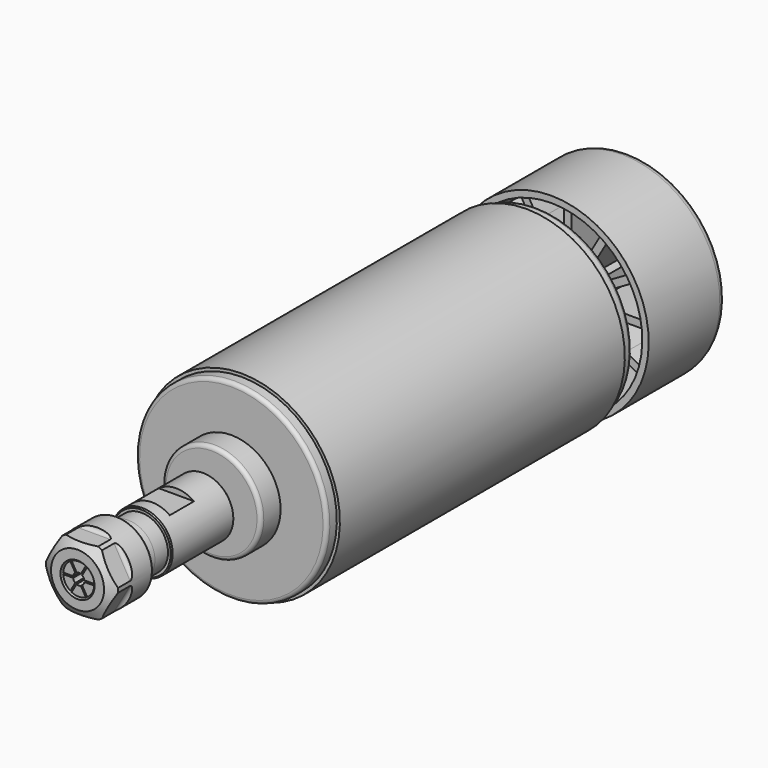
from build123d import *

# Parameters (mm, degrees)
F0_W      = 2.5
F0_H      = 4
F2_R      = 2
F3_R      = 1
F4_SIZE   = 1
F6_W      = 8
F6_H      = 2.5
F7_DEPTH  = 12.5
F10_R     = 0.5
F13_R     = 12
F14_DEPTH = 6.5
F15_R     = 0.99999
F16_R     = 4.5
F17_DEPTH = 0.4
F18_R     = 4.5
F19_DEPTH = 3
F21_DEPTH = 20
F23_DEPTH = 16.5


# Not quite as in the source:
# - a fillet or chamfer that OpenCascade refuses, or shapes differently, is made with other operations: its cross-section is extruded or revolved along the edge and cut away or added
# - a fillet or chamfer is up to 0.001 mm smaller than in the source, because OpenCascade refuses the exact size


with BuildPart() as f1:
    # F0 (on Right) → F1 (revolve)
    with BuildSketch(Plane.YZ):
        Polygon((-68.75, 4), (-68.75, 0), (68.75, 0), (68.75, 4), (65.25, 4), (65.25, 17.25), (68.75, 17.25), (68.75, 25.75), (43.29, 25.75), (43.29, 24.05), (48.75, 24.05), (48.75, 4), (44.93, 4), (44.93, 13), (38.39, 13), (38.39, 25.2), (35.09, 25.2), (35.09, 26), (-58.91, 26), (-58.91, 25.2), (-62.21, 25.2), (-62.21, 13), (-68.75, 13), align=None)
        with Locations((-70, 2)):
            Rectangle(F0_W, F0_H)
        Polygon((-106.25, 0), (-71.25, 0), (-71.25, 4), (-71.25, 8), (-91.85, 8), (-91.85, 7), (-96.15, 7), (-106.25, 6.75), align=None)
    revolve(axis=Axis((0, -2.606525797, 0), (0, 1, 0)))

    # F2
    f2_edges = [f1.edges().sort_by_distance(p)[0] for p in [
        (0, 68.75, -25.75),
    ]]
    fillet(f2_edges, radius=F2_R)

    # F3
    f3_edges = [f1.edges().sort_by_distance(p)[0] for p in [
        (0, 38.39, -25.2),
        (0, -62.21, -25.2),
        (0, -68.75, -13),
        (0, 44.93, -13),
    ]]
    fillet(f3_edges, radius=F3_R)

    # F4
    f4_edges = [f1.edges().sort_by_distance(p)[0] for p in [
        (0, 68.75, -4),
    ]]
    chamfer(f4_edges, length=F4_SIZE)

    # F5: chamfer of 0.3 on 3 edges, made by hand

    # F5_s1 → F5_t2 (revolve, cut)
    with BuildSketch(Plane.YZ):
        Polygon((-71.25, 7.7), (-71.55, 8), (-71.25, 8), align=None)
    revolve(axis=Axis((0, -71.25, 0), (0, 1, 0)), mode=Mode.SUBTRACT)

    # F5_s3 → F5_t4 (revolve, cut)
    with BuildSketch(Plane.YZ):
        Polygon((-91.55, 8), (-91.85, 7.7), (-91.85, 8), align=None)
    revolve(axis=Axis((0, -91.85, 0), (0, 1, 0)), mode=Mode.SUBTRACT)

    # F5_s5 → F5_t6 (revolve, cut)
    with BuildSketch(Plane.YZ):
        Polygon((-105.9574234688, 6.7572419933), (-106.25, 6.4573338539), (-106.25, 6.75), align=None)
    revolve(axis=Axis((0, -106.25, 0), (0, 1, 0)), mode=Mode.SUBTRACT)

    # F6 (on Right) → F7 (cut, symmetric)
    with BuildSketch(Plane.YZ):
        with Locations((-84.35, 7.75)):
            Rectangle(F6_W, F6_H)
        with Locations((-84.35, -7.75)):
            Rectangle(F6_W, F6_H)
    extrude(amount=F7_DEPTH, both=True, mode=Mode.SUBTRACT)

    # F20 (on face) → F21 (cut)
    with BuildSketch(Plane(origin=(0, 65.25, 0), x_dir=(-1, 0, 0), z_dir=(0, 1, 0))):
        with BuildLine():
            ThreePointArc((-5.5, 4.3301270189), (-4.9497474683, 4.9497474683), (-4.3301270189, 5.5))
            Line((-4.3301270189, 5.5), (-9.4765204534, 14.4138149043))
            ThreePointArc((-9.4765204534, 14.4138149043), (-12.1975919755, 12.1975919755), (-14.4138149043, 9.4765204534))
            Line((-14.4138149043, 9.4765204534), (-5.5, 4.3301270189))
        make_face()
        with BuildLine():
            Line((-1, 6.9282032303), (-1, 17.2209900993))
            ThreePointArc((-1, 17.2209900993), (-4.464628528, 16.6622205035), (-7.7444696459, 15.4138149043))
            Line((-7.7444696459, 15.4138149043), (-2.5980762114, 6.5))
            ThreePointArc((-2.5980762114, 6.5), (-1.8117333157, 6.761480784), (-1, 6.9282032303))
        make_face()
        with BuildLine():
            ThreePointArc((7.7444696459, 15.4138149043), (4.464628528, 16.6622205035), (1, 17.2209900993))
            Line((1, 17.2209900993), (1, 6.9282032303))
            ThreePointArc((1, 6.9282032303), (1.8117333157, 6.761480784), (2.5980762114, 6.5))
            Line((2.5980762114, 6.5), (7.7444696459, 15.4138149043))
        make_face()
        with BuildLine():
            Line((-6.5, 2.5980762114), (-15.4138149043, 7.7444696459))
            ThreePointArc((-15.4138149043, 7.7444696459), (-16.6622205035, 4.464628528), (-17.2209900993, 1))
            Line((-17.2209900993, 1), (-6.9282032303, 1))
            ThreePointArc((-6.9282032303, 1), (-6.761480784, 1.8117333157), (-6.5, 2.5980762114))
        make_face()
        with BuildLine():
            Line((-6.9282032303, -1), (-17.2209900993, -1))
            ThreePointArc((-17.2209900993, -1), (-16.6622205035, -4.464628528), (-15.4138149043, -7.7444696459))
            Line((-15.4138149043, -7.7444696459), (-6.5, -2.5980762114))
            ThreePointArc((-6.5, -2.5980762114), (-6.761480784, -1.8117333157), (-6.9282032303, -1))
        make_face()
        with BuildLine():
            Line((-5.5, -4.3301270189), (-14.4138149043, -9.4765204534))
            ThreePointArc((-14.4138149043, -9.4765204534), (-12.1975919755, -12.1975919755), (-9.4765204534, -14.4138149043))
            Line((-9.4765204534, -14.4138149043), (-4.3301270189, -5.5))
            ThreePointArc((-4.3301270189, -5.5), (-4.9497474683, -4.9497474683), (-5.5, -4.3301270189))
        make_face()
        with BuildLine():
            Line((-2.5980762114, -6.5), (-7.7444696459, -15.4138149043))
            ThreePointArc((-7.7444696459, -15.4138149043), (-4.464628528, -16.6622205035), (-1, -17.2209900993))
            Line((-1, -17.2209900993), (-1, -6.9282032303))
            ThreePointArc((-1, -6.9282032303), (-1.8117333157, -6.761480784), (-2.5980762114, -6.5))
        make_face()
        with BuildLine():
            Line((1, -6.9282032303), (1, -17.2209900993))
            ThreePointArc((1, -17.2209900993), (4.464628528, -16.6622205035), (7.7444696459, -15.4138149043))
            Line((7.7444696459, -15.4138149043), (2.5980762114, -6.5))
            ThreePointArc((2.5980762114, -6.5), (1.8117333157, -6.761480784), (1, -6.9282032303))
        make_face()
        with BuildLine():
            Line((4.3301270189, -5.5), (9.4765204534, -14.4138149043))
            ThreePointArc((9.4765204534, -14.4138149043), (12.1975919755, -12.1975919755), (14.4138149043, -9.4765204534))
            Line((14.4138149043, -9.4765204534), (5.5, -4.3301270189))
            ThreePointArc((5.5, -4.3301270189), (4.9497474683, -4.9497474683), (4.3301270189, -5.5))
        make_face()
        with BuildLine():
            Line((6.5, -2.5980762114), (15.4138149043, -7.7444696459))
            ThreePointArc((15.4138149043, -7.7444696459), (16.6622205035, -4.464628528), (17.2209900993, -1))
            Line((17.2209900993, -1), (6.9282032303, -1))
            ThreePointArc((6.9282032303, -1), (6.761480784, -1.8117333157), (6.5, -2.5980762114))
        make_face()
        with BuildLine():
            Line((6.9282032303, 1), (17.2209900993, 1))
            ThreePointArc((17.2209900993, 1), (16.6622205035, 4.464628528), (15.4138149043, 7.7444696459))
            Line((15.4138149043, 7.7444696459), (6.5, 2.5980762114))
            ThreePointArc((6.5, 2.5980762114), (6.761480784, 1.8117333157), (6.9282032303, 1))
        make_face()
        with BuildLine():
            Line((5.5, 4.3301270189), (14.4138149043, 9.4765204534))
            ThreePointArc((14.4138149043, 9.4765204534), (12.1975919755, 12.1975919755), (9.4765204534, 14.4138149043))
            Line((9.4765204534, 14.4138149043), (4.3301270189, 5.5))
            ThreePointArc((4.3301270189, 5.5), (4.9497474683, 4.9497474683), (5.5, 4.3301270189))
        make_face()
    extrude(amount=-F21_DEPTH, mode=Mode.SUBTRACT)

    # F22 (on face) → F23 (cut)
    with BuildSketch(Plane.XZ.offset(-48.75)):
        with BuildLine():
            Line((17.2209900993, 1), (24.0292009855, 1))
            ThreePointArc((24.0292009855, 1), (23.2305161223, 6.2245980347), (21.3098984861, 11.1485750889))
            Line((21.3098984861, 11.1485750889), (15.4138149043, 7.7444696459))
            ThreePointArc((15.4138149043, 7.7444696459), (16.6622205035, 4.464628528), (17.2209900993, 1))
        make_face()
        with BuildLine():
            ThreePointArc((21.3098984861, -11.1485750889), (23.2305161223, -6.2245980347), (24.0292009855, -1))
            Line((24.0292009855, -1), (17.2209900993, -1))
            ThreePointArc((17.2209900993, -1), (16.6622205035, -4.464628528), (15.4138149043, -7.7444696459))
            Line((15.4138149043, -7.7444696459), (21.3098984861, -11.1485750889))
        make_face()
        with BuildLine():
            Line((14.4138149043, 9.4765204534), (20.3098984861, 12.8806258965))
            ThreePointArc((20.3098984861, 12.8806258965), (17.0059180875, 17.0059180875), (12.8806258965, 20.3098984861))
            Line((12.8806258965, 20.3098984861), (9.4765204534, 14.4138149043))
            ThreePointArc((9.4765204534, 14.4138149043), (12.1975919755, 12.1975919755), (14.4138149043, 9.4765204534))
        make_face()
        with BuildLine():
            ThreePointArc((12.8806258965, -20.3098984861), (17.0059180875, -17.0059180875), (20.3098984861, -12.8806258965))
            Line((20.3098984861, -12.8806258965), (14.4138149043, -9.4765204534))
            ThreePointArc((14.4138149043, -9.4765204534), (12.1975919755, -12.1975919755), (9.4765204534, -14.4138149043))
            Line((9.4765204534, -14.4138149043), (12.8806258965, -20.3098984861))
        make_face()
        with BuildLine():
            Line((7.7444696459, 15.4138149043), (11.1485750889, 21.3098984861))
            ThreePointArc((11.1485750889, 21.3098984861), (6.2245980347, 23.2305161223), (1, 24.0292009855))
            Line((1, 24.0292009855), (1, 17.2209900993))
            ThreePointArc((1, 17.2209900993), (4.464628528, 16.6622205035), (7.7444696459, 15.4138149043))
        make_face()
        with BuildLine():
            ThreePointArc((1, -24.0292009855), (6.2245980347, -23.2305161223), (11.1485750889, -21.3098984861))
            Line((11.1485750889, -21.3098984861), (7.7444696459, -15.4138149043))
            ThreePointArc((7.7444696459, -15.4138149043), (4.464628528, -16.6622205035), (1, -17.2209900993))
            Line((1, -17.2209900993), (1, -24.0292009855))
        make_face()
        with BuildLine():
            ThreePointArc((1, -17.2209900993), (4.464628528, -16.6622205035), (7.7444696459, -15.4138149043))
            Line((7.7444696459, -15.4138149043), (2.5980762114, -6.5))
            ThreePointArc((2.5980762114, -6.5), (1.8117333157, -6.761480784), (1, -6.9282032303))
            Line((1, -6.9282032303), (1, -17.2209900993))
        make_face()
        with BuildLine():
            Line((-1, 17.2209900993), (-1, 24.0292009855))
            ThreePointArc((-1, 24.0292009855), (-6.2245980347, 23.2305161223), (-11.1485750889, 21.3098984861))
            Line((-11.1485750889, 21.3098984861), (-7.7444696459, 15.4138149043))
            ThreePointArc((-7.7444696459, 15.4138149043), (-4.464628528, 16.6622205035), (-1, 17.2209900993))
        make_face()
        with BuildLine():
            ThreePointArc((-11.1485750889, -21.3098984861), (-6.2245980347, -23.2305161223), (-1, -24.0292009855))
            Line((-1, -24.0292009855), (-1, -17.2209900993))
            ThreePointArc((-1, -17.2209900993), (-4.464628528, -16.6622205035), (-7.7444696459, -15.4138149043))
            Line((-7.7444696459, -15.4138149043), (-11.1485750889, -21.3098984861))
        make_face()
        with BuildLine():
            Line((-1, 6.9282032303), (-1, 17.2209900993))
            ThreePointArc((-1, 17.2209900993), (-4.464628528, 16.6622205035), (-7.7444696459, 15.4138149043))
            Line((-7.7444696459, 15.4138149043), (-2.5980762114, 6.5))
            ThreePointArc((-2.5980762114, 6.5), (-1.8117333157, 6.761480784), (-1, 6.9282032303))
        make_face()
        with BuildLine():
            ThreePointArc((-7.7444696459, -15.4138149043), (-4.464628528, -16.6622205035), (-1, -17.2209900993))
            Line((-1, -17.2209900993), (-1, -6.9282032303))
            ThreePointArc((-1, -6.9282032303), (-1.8117333157, -6.761480784), (-2.5980762114, -6.5))
            Line((-2.5980762114, -6.5), (-7.7444696459, -15.4138149043))
        make_face()
        with BuildLine():
            Line((-9.4765204534, 14.4138149043), (-12.8806258965, 20.3098984861))
            ThreePointArc((-12.8806258965, 20.3098984861), (-17.0059180875, 17.0059180875), (-20.3098984861, 12.8806258965))
            Line((-20.3098984861, 12.8806258965), (-14.4138149043, 9.4765204534))
            ThreePointArc((-14.4138149043, 9.4765204534), (-12.1975919755, 12.1975919755), (-9.4765204534, 14.4138149043))
        make_face()
        with BuildLine():
            ThreePointArc((-20.3098984861, -12.8806258965), (-17.0059180875, -17.0059180875), (-12.8806258965, -20.3098984861))
            Line((-12.8806258965, -20.3098984861), (-9.4765204534, -14.4138149043))
            ThreePointArc((-9.4765204534, -14.4138149043), (-12.1975919755, -12.1975919755), (-14.4138149043, -9.4765204534))
            Line((-14.4138149043, -9.4765204534), (-20.3098984861, -12.8806258965))
        make_face()
        with BuildLine():
            Line((-4.3301270189, 5.5), (-9.4765204534, 14.4138149043))
            ThreePointArc((-9.4765204534, 14.4138149043), (-12.1975919755, 12.1975919755), (-14.4138149043, 9.4765204534))
            Line((-14.4138149043, 9.4765204534), (-5.5, 4.3301270189))
            ThreePointArc((-5.5, 4.3301270189), (-4.9497474683, 4.9497474683), (-4.3301270189, 5.5))
        make_face()
        with BuildLine():
            ThreePointArc((-14.4138149043, -9.4765204534), (-12.1975919755, -12.1975919755), (-9.4765204534, -14.4138149043))
            Line((-9.4765204534, -14.4138149043), (-4.3301270189, -5.5))
            ThreePointArc((-4.3301270189, -5.5), (-4.9497474683, -4.9497474683), (-5.5, -4.3301270189))
            Line((-5.5, -4.3301270189), (-14.4138149043, -9.4765204534))
        make_face()
        with BuildLine():
            Line((-15.4138149043, 7.7444696459), (-21.3098984861, 11.1485750889))
            ThreePointArc((-21.3098984861, 11.1485750889), (-23.2305161223, 6.2245980347), (-24.0292009855, 1))
            Line((-24.0292009855, 1), (-17.2209900993, 1))
            ThreePointArc((-17.2209900993, 1), (-16.6622205035, 4.464628528), (-15.4138149043, 7.7444696459))
        make_face()
        with BuildLine():
            ThreePointArc((-24.0292009855, -1), (-23.2305161223, -6.2245980347), (-21.3098984861, -11.1485750889))
            Line((-21.3098984861, -11.1485750889), (-15.4138149043, -7.7444696459))
            ThreePointArc((-15.4138149043, -7.7444696459), (-16.6622205035, -4.464628528), (-17.2209900993, -1))
            Line((-17.2209900993, -1), (-24.0292009855, -1))
        make_face()
        with BuildLine():
            Line((-6.5, 2.5980762114), (-15.4138149043, 7.7444696459))
            ThreePointArc((-15.4138149043, 7.7444696459), (-16.6622205035, 4.464628528), (-17.2209900993, 1))
            Line((-17.2209900993, 1), (-6.9282032303, 1))
            ThreePointArc((-6.9282032303, 1), (-6.761480784, 1.8117333157), (-6.5, 2.5980762114))
        make_face()
        with BuildLine():
            ThreePointArc((-17.2209900993, -1), (-16.6622205035, -4.464628528), (-15.4138149043, -7.7444696459))
            Line((-15.4138149043, -7.7444696459), (-6.5, -2.5980762114))
            ThreePointArc((-6.5, -2.5980762114), (-6.761480784, -1.8117333157), (-6.9282032303, -1))
            Line((-6.9282032303, -1), (-17.2209900993, -1))
        make_face()
    extrude(amount=-F23_DEPTH, mode=Mode.SUBTRACT)


with BuildPart() as f9:
    # F8 (on Right) → F9 (revolve)
    with BuildSketch(Plane.YZ):
        Polygon((-112.95, 0), (-106.4195036888, 0), (-106.4195036888, 6.8374252878), (-99.95, 7.0293229073), (-99.95, 9.5), (-112.95, 9.5), align=None)
    revolve(axis=Axis((0, -49.975, 0), (0, -1, 0)))

    # F10
    f10_edges = [f9.edges().sort_by_distance(p)[0] for p in [
        (0, -99.95, -9.5),
    ]]
    fillet(f10_edges, radius=F10_R)

    # F11 (on Right) → F12 (revolve, cut)
    with BuildSketch(Plane.YZ):
        Polygon((-112.95, 9.5), (-112.95, 7), (-111.45, 9.5), align=None)
    revolve(axis=Axis((0, -60.4325269299, 0), (0, -1, 0)), mode=Mode.SUBTRACT)

    # F13 (on face) → F14 (cut)
    with BuildSketch(Plane.XZ.offset(112.95)):
        Circle(F13_R)
        Polygon((-9.8149545762, 0), (-4.9074772881, 8.5), (4.9074772881, 8.5), (9.8149545762, 0), (4.9074772881, -8.5), (-4.9074772881, -8.5), align=None, mode=Mode.SUBTRACT)
    extrude(amount=-F14_DEPTH, mode=Mode.SUBTRACT)

    # F15 (radius 1 in the source; OpenCascade refuses exactly that, so slightly less here)
    f15_edges = [f9.edges().sort_by_distance(p)[0] for p in [
        (0, -106.45, 8.5),
        (7.361216, -106.45, 4.25),
        (7.361216, -106.45, -4.25),
        (0, -106.45, -8.5),
        (-7.361216, -106.45, -4.25),
        (-7.361216, -106.45, 4.25),
    ]]
    fillet(f15_edges, radius=F15_R)

    # F16 (on face) → F17 (cut)
    with BuildSketch(Plane.XZ.offset(112.95)):
        Circle(F16_R)
    extrude(amount=-F17_DEPTH, mode=Mode.SUBTRACT)

    # F18 (on face) → F19 (cut)
    with BuildSketch(Plane.XZ.offset(112.55)):
        Circle(F18_R)
        with BuildLine():
            ThreePointArc((-2.2207646037, -3.4464771253), (-3.5507041555, -2.05), (-4.0951190459, -0.2))
            Line((-4.0951190459, -0.2), (-1.4866068747, -0.2))
            ThreePointArc((-1.4866068747, -0.2), (-1.2990381057, -0.75), (-0.9165085181, -1.187439319))
            Line((-0.9165085181, -1.187439319), (-2.2207646037, -3.4464771253))
        make_face(mode=Mode.SUBTRACT)
        with BuildLine():
            ThreePointArc((1.8743544422, -3.6464771253), (0, -4.1), (-1.8743544422, -3.6464771253))
            Line((-1.8743544422, -3.6464771253), (-0.5700983566, -1.387439319))
            ThreePointArc((-0.5700983566, -1.387439319), (0, -1.5), (0.5700983566, -1.387439319))
            Line((0.5700983566, -1.387439319), (1.8743544422, -3.6464771253))
        make_face(mode=Mode.SUBTRACT)
        with BuildLine():
            ThreePointArc((4.0951190459, -0.2), (3.5507041555, -2.05), (2.2207646037, -3.4464771253))
            Line((2.2207646037, -3.4464771253), (0.9165085181, -1.187439319))
            ThreePointArc((0.9165085181, -1.187439319), (1.2990381057, -0.75), (1.4866068747, -0.2))
            Line((1.4866068747, -0.2), (4.0951190459, -0.2))
        make_face(mode=Mode.SUBTRACT)
        with BuildLine():
            Line((-2.2207646037, 3.4464771253), (-0.9165085181, 1.187439319))
            ThreePointArc((-0.9165085181, 1.187439319), (-1.2990381057, 0.75), (-1.4866068747, 0.2))
            Line((-1.4866068747, 0.2), (-4.0951190459, 0.2))
            ThreePointArc((-4.0951190459, 0.2), (-3.5507041555, 2.05), (-2.2207646037, 3.4464771253))
        make_face(mode=Mode.SUBTRACT)
        with BuildLine():
            Line((-0.5700983566, 1.387439319), (-1.8743544422, 3.6464771253))
            ThreePointArc((-1.8743544422, 3.6464771253), (0, 4.1), (1.8743544422, 3.6464771253))
            Line((1.8743544422, 3.6464771253), (0.5700983566, 1.387439319))
            ThreePointArc((0.5700983566, 1.387439319), (0, 1.5), (-0.5700983566, 1.387439319))
        make_face(mode=Mode.SUBTRACT)
        with BuildLine():
            ThreePointArc((2.2207646037, 3.4464771253), (3.5507041555, 2.05), (4.0951190459, 0.2))
            Line((4.0951190459, 0.2), (1.4866068747, 0.2))
            ThreePointArc((1.4866068747, 0.2), (1.2990381057, 0.75), (0.9165085181, 1.187439319))
            Line((0.9165085181, 1.187439319), (2.2207646037, 3.4464771253))
        make_face(mode=Mode.SUBTRACT)
    extrude(amount=-F19_DEPTH, mode=Mode.SUBTRACT)


solid = Compound([f1.part, f9.part])
